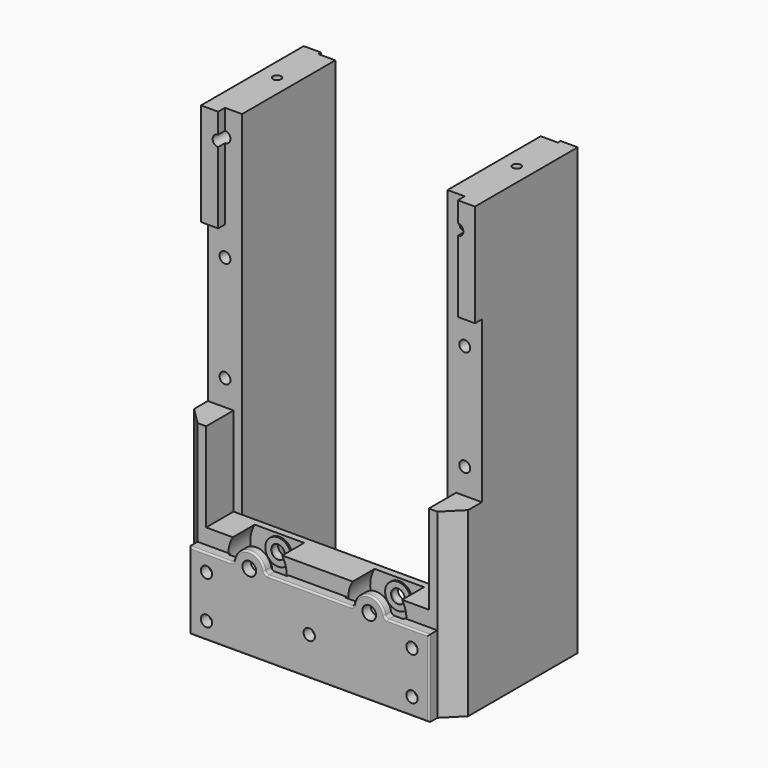
from build123d import *

# Parameters (mm, degrees)
F2_DEPTH         = 27
F4_DEPTH         = 26
F6_DEPTH         = 47
F8_DEPTH         = 30
F9_R             = 8.5
F10_DEPTH        = 8
F11_R            = 3.75
F11_R_2          = 2
F12_DEPTH        = 0.5
F13_DEPTH        = 25
F14_SIZE         = 5
F15_R            = 2
F16_DEPTH        = 3
F18_R            = 8.5
F18_R_2          = 3.75
F19_DEPTH        = 0.5
F21_D            = 3.2
F21_DEPTH        = 8
F21_TIP          = 0.9613769904
F24_D            = 3.2
F24_DEPTH        = 8
F24_TIP          = 0.9613769904
F24_ON_F22_D     = 3.2
F24_ON_F22_DEPTH = 8
F24_ON_F22_TIP   = 0.9613769904
F25_R            = 1
F26_R            = 0.5
F27_D            = 3.3
F28_D            = 2.4
F28_DEPTH        = 8
F28_TIP          = 0.7210327428
F30_D            = 2.4
F30_DEPTH        = 2.5
F30_TIP          = 0.7210327428


# Not quite as in the source:
# - a feature names something its author has since deleted; it is built from what else it names


with BuildPart() as f2:
    # F1 (on offset) → F2 (new body)
    with BuildSketch(Plane.XY.offset(-90)):
        Polygon((30, -14.782029699), (-30, -14.782029699), (-30, 19.217970301), (-35, 19.217970301), (-35, 20.217970301), (-40, 20.217970301), (-40, -24.782029699), (40, -24.782029699), (40, 20.217970301), (35, 20.217970301), (35, 19.217970301), (30, 19.217970301), align=None)
    extrude(amount=F2_DEPTH)

    # F3 (on face) → F4 (join)
    with BuildSketch(Plane.XY.offset(-63)):
        Polygon((-32.5, -14.782029699), (-30, -14.782029699), (-30, 19.217970301), (-35, 19.217970301), (-35, 20.217970301), (-40, 20.217970301), (-40, -24.782029699), (-32.5, -24.782029699), align=None)
        Polygon((40, -24.782029699), (40, 20.217970301), (35, 20.217970301), (35, 19.217970301), (30, 19.217970301), (30, -14.782029699), (32.5, -14.782029699), (32.5, -24.782029699), align=None)
    extrude(amount=F4_DEPTH)

    # F5 (on face) → F6 (join)
    with BuildSketch(Plane.XY.offset(-37)):
        Polygon((40, -14.782029699), (40, 20.217970301), (35, 20.217970301), (35, 19.217970301), (30, 19.217970301), (30, -14.782029699), align=None)
        Polygon((-35, 20.217970301), (-40, 20.217970301), (-40, -14.782029699), (-30, -14.782029699), (-30, 19.217970301), (-35, 19.217970301), align=None)
    extrude(amount=F6_DEPTH)

    # F7 (on face) → F8 (join)
    with BuildSketch(Plane.XY.offset(10)):
        Polygon((40, -17.282029699), (40, 20.217970301), (35, 20.217970301), (35, 19.217970301), (30, 19.217970301), (30, -14.782029699), (35, -14.782029699), (35, -17.282029699), align=None)
        Polygon((-30, 19.217970301), (-35, 19.217970301), (-35, 20.217970301), (-40, 20.217970301), (-40, -17.282029699), (-35, -17.282029699), (-35, -14.782029699), (-30, -14.782029699), align=None)
    extrude(amount=F8_DEPTH)

    # F9 (on face) → F10 (cut)
    with BuildSketch(Plane.XZ.offset(24.782029699)):
        with Locations((17.5, -67.5)):
            Circle(F9_R)
        with Locations((-17.5, -67.5)):
            Circle(F9_R)
    extrude(amount=-F10_DEPTH, mode=Mode.SUBTRACT)

    # F11 (on face) → F12 (join)
    with BuildSketch(Plane.XZ.offset(16.782029699)):
        with Locations((17.5, -67.5)):
            Circle(F11_R)
        with Locations((17.5, -67.5)):
            Circle(F11_R_2, mode=Mode.SUBTRACT)
        with Locations((-17.5, -67.5)):
            Circle(F11_R)
        with Locations((-17.5, -67.5)):
            Circle(F11_R_2, mode=Mode.SUBTRACT)
    extrude(amount=F12_DEPTH)

    # F13 (cut): faces of the model
    f13_faces = [f2.faces().sort_by_distance(p)[0] for p in [
        (17.5, -16.782029699, -67.5),
        (-17.5, -16.782029699, -67.5),
    ]]
    extrude(f13_faces, amount=-F13_DEPTH, mode=Mode.SUBTRACT)

    # F14
    f14_edges = [f2.edges().sort_by_distance(p)[0] for p in [
        (40, -24.78203, -63.5),
        (-40, -24.78203, -63.5),
    ]]
    chamfer(f14_edges, length=F14_SIZE)

    # F21 (one way)
    with BuildSketch(Plane(origin=(0, 20.217970301, 0), x_dir=(-1, 0, 0), z_dir=(0, 1, 0))):
        with Locations((35, 32.5), (35, -25), (-35, -25), (-35, 32.5), (-35, -82.5), (35, -82.5)):
            Circle(F21_D / 2)
    extrude(amount=-F21_DEPTH, mode=Mode.SUBTRACT)
    with Locations(Plane(origin=(0, 20.217970301, 0), x_dir=(-1, 0, 0), z_dir=(0, 1, 0))):
        with Locations((35, 32.5), (35, -25), (-35, -25), (-35, 32.5), (-35, -82.5), (35, -82.5)):
            with Locations((0, 0, -(F21_DEPTH + F21_TIP / 2))):  # 118° drill point
                Cone(0, F21_D / 2, F21_TIP, mode=Mode.SUBTRACT)

    # F24 (one way)
    with BuildSketch(Plane.XZ.offset(17.282029699)):
        with Locations((-35, 32.5), (35, 32.5)):
            Circle(F24_D / 2)
    extrude(amount=-F24_DEPTH, mode=Mode.SUBTRACT)
    with Locations(Plane.XZ.offset(17.282029699)):
        with Locations((-35, 32.5), (35, 32.5)):
            with Locations((0, 0, -(F24_DEPTH + F24_TIP / 2))):  # 118° drill point
                Cone(0, F24_D / 2, F24_TIP, mode=Mode.SUBTRACT)

    # F24 on F22 (one way)
    with BuildSketch(Plane.XZ.offset(14.782029699)):
        with Locations((-35, 1.5), (35, 1.5), (-35, -29.5), (35, -29.5)):
            Circle(F24_ON_F22_D / 2)
    extrude(amount=-F24_ON_F22_DEPTH, mode=Mode.SUBTRACT)
    with Locations(Plane.XZ.offset(14.782029699)):
        with Locations((-35, 1.5), (35, 1.5), (-35, -29.5), (35, -29.5)):
            with Locations((0, 0, -(F24_ON_F22_DEPTH + F24_ON_F22_TIP / 2))):  # 118° drill point
                Cone(0, F24_ON_F22_D / 2, F24_ON_F22_TIP, mode=Mode.SUBTRACT)

    # F28 (one way)
    with BuildSketch(Plane.XZ.offset(27.782029699)):
        with Locations((-30, -72.5), (-30, -85), (0, -78.75), (30, -72.5), (30, -85)):
            Circle(F28_D / 2)
    extrude(amount=-F28_DEPTH, mode=Mode.SUBTRACT)
    with Locations(Plane.XZ.offset(27.782029699)):
        with Locations((-30, -72.5), (-30, -85), (0, -78.75), (30, -72.5), (30, -85)):
            with Locations((0, 0, -(F28_DEPTH + F28_TIP / 2))):  # 118° drill point
                Cone(0, F28_D / 2, F28_TIP, mode=Mode.SUBTRACT)

    # F30
    with Locations(Plane.XY.offset(40)):
        with Locations((-35, 4.217970301), (35, 4.217970301)):
            Hole(F30_D / 2, depth=F30_DEPTH)
            with Locations((0, 0, -(F30_DEPTH + F30_TIP / 2))):  # 118° drill point
                Cone(0, F30_D / 2, F30_TIP, mode=Mode.SUBTRACT)


with BuildPart() as f16:
    # F15 (on face) → F16 (new body)
    with BuildSketch(Plane.XZ.offset(24.782029699)):
        with BuildLine():
            Line((35, -67.5), (22, -67.5))
            ThreePointArc((22, -67.5), (17.5, -63), (13, -67.5))
            Line((13, -67.5), (-13, -67.5))
            ThreePointArc((-13, -67.5), (-17.5, -63), (-22, -67.5))
            Line((-22, -67.5), (-35, -67.5))
            Line((-35, -67.5), (-35, -90))
            Line((-35, -90), (35, -90))
            Line((35, -90), (35, -67.5))
        make_face()
        with Locations((-17.5, -67.5)):
            Circle(F15_R, mode=Mode.SUBTRACT)
        with Locations((17.5, -67.5)):
            Circle(F15_R, mode=Mode.SUBTRACT)
    extrude(amount=F16_DEPTH)

    # F18 (on face) → F19 (cut)
    with BuildSketch(Plane.XZ.offset(24.782029699)):
        with Locations((17, -67.5)):
            Circle(F18_R)
        with Locations((17, -67.5)):
            Circle(F18_R_2, mode=Mode.SUBTRACT)
        with Locations((-17, -67.5)):
            Circle(F18_R)
        with Locations((-17, -67.5)):
            Circle(F18_R_2, mode=Mode.SUBTRACT)
    extrude(amount=F19_DEPTH, mode=Mode.SUBTRACT)

    # F25
    f25_edges = [f16.edges().sort_by_distance(p)[0] for p in [
        (-13, -26.53203, -67.5),
        (22, -26.53203, -67.5),
        (13, -26.53203, -67.5),
        (-22, -26.53203, -67.5),
    ]]
    fillet(f25_edges, radius=F25_R)

    # F26
    f26_edges = [f16.edges().sort_by_distance(p)[0] for p in [
        (-28.954163, -27.78203, -67.5),
        (-22.268725, -27.78203, -67.268706),
        (-17.5, -27.78203, -63),
        (-12.731275, -27.78203, -67.268706),
        (35, -27.78203, -78.75),
        (0, -27.78203, -90),
        (-35, -27.78203, -78.75),
        (28.954163, -27.78203, -67.5),
        (22.268725, -27.78203, -67.268706),
        (17.5, -27.78203, -63),
        (12.731275, -27.78203, -67.268706),
        (0, -27.78203, -67.5),
    ]]
    fillet(f26_edges, radius=F26_R)

    # F27 (through all)
    with Locations(Plane.XZ.offset(27.782029699)):
        with Locations((30, -72.5), (0, -78.75), (30, -85), (-30, -85), (-30, -72.5)):
            Hole(F27_D / 2)


solid = Compound([f2.part, f16.part])
